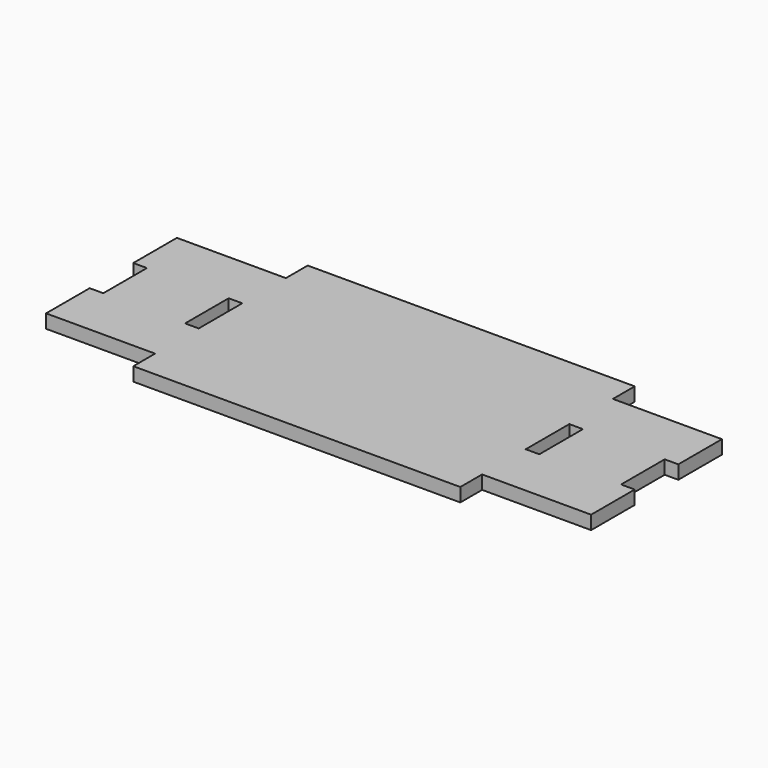
from build123d import *

# Parameters (mm, degrees)
F0_W     = 3.175
F0_H     = 12.7
F1_DEPTH = 3.175


# Not quite as in the source:
# - a feature names something its author has since deleted; it is built from what else it names


with BuildPart() as f1:
    # F0 (on Top) → F1 (new body)
    with BuildSketch(Plane.XY):
        Polygon((38.1, 19.05), (38.1, 25.4), (-38.1, 25.4), (-38.1, 19.05), (-63.5, 19.05), (-63.5, 6.35), (-60.325, 6.35), (-60.325, -6.35), (-63.5, -6.35), (-63.5, -19.05), (-38.1, -19.05), (-38.1, -25.4), (38.1, -25.4), (38.1, -19.05), (63.5, -19.05), (63.5, -6.35), (60.325, -6.35), (60.325, 6.35), (63.5, 6.35), (63.5, 19.05), align=None)
        with Locations((-39.6875, 0)):
            Rectangle(F0_W, F0_H, mode=Mode.SUBTRACT)
        with Locations((39.6875, 0)):
            Rectangle(F0_W, F0_H, mode=Mode.SUBTRACT)
    extrude(amount=F1_DEPTH)


solid = f1.part
